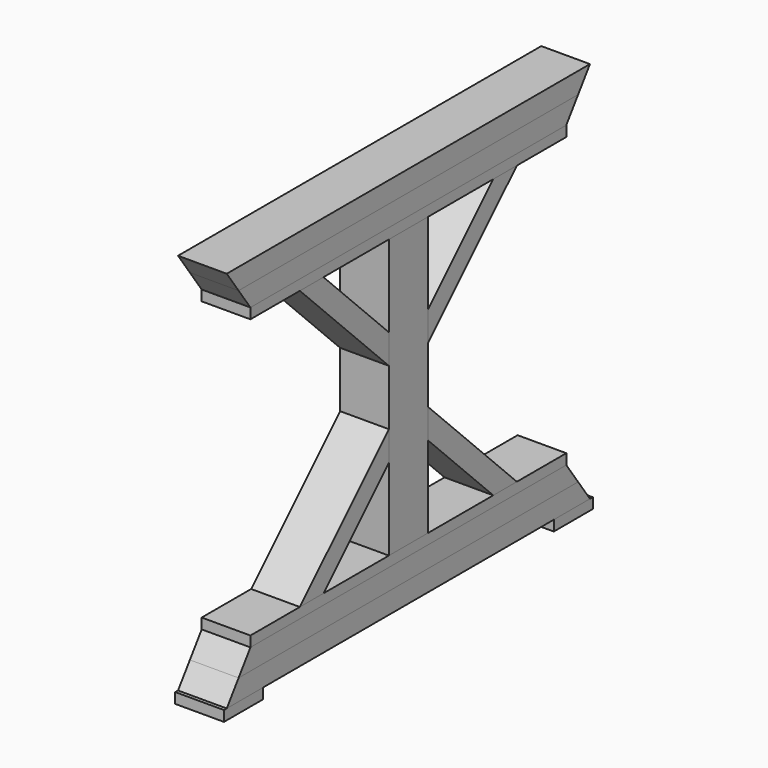
from build123d import *

# Parameters (mm, degrees)
F0_W      = 88.9
F0_H      = 38.1
F1_DEPTH  = 414.3375
F2_W      = 88.9
F2_H      = 38.1
F3_DEPTH  = 414.3375
F5_W      = 88.9
F5_H      = 19.05
F6_DEPTH  = 88.9
F8_W      = 88.9
F8_H      = 19.05
F9_DEPTH  = 360.3625
F11_DEPTH = 88.901
F12_W     = 88.9
F12_H     = 88.9
F13_DEPTH = 508
F17_DEPTH = 88.9


# Not quite as in the source:
# - a feature names something its author has since deleted; it is built from what else it names


with BuildPart() as f1:
    # F0 (on Front) → F1 (new body, symmetric)
    with BuildSketch(Plane.XZ):
        with Locations((44.45, 19.05)):
            Rectangle(F0_W, F0_H)
    extrude(amount=F1_DEPTH, both=True)


with BuildPart() as f3:
    # F2 (on Front) → F3 (new body, symmetric)
    with BuildSketch(Plane.XZ):
        with Locations((44.45, 57.15)):
            Rectangle(F2_W, F2_H)
    extrude(amount=F3_DEPTH, both=True)


with BuildPart() as f6:
    # F5 (on offset) → F6 (new body)
    with BuildSketch(Plane.XZ.offset(420.6875)):
        with Locations((44.45, -9.525)):
            Rectangle(F5_W, F5_H)
    extrude(amount=-F6_DEPTH)


with BuildPart() as f7_1:
    # F7: instance of F6
    add(f6.part.mirror(Plane.XZ))


with BuildPart() as f9:
    # F8 (on Front) → F9 (new body, symmetric)
    with BuildSketch(Plane.XZ):
        with Locations((44.45, 85.725)):
            Rectangle(F8_W, F8_H)
    extrude(amount=F9_DEPTH, both=True)


with BuildPart() as f11_tool:
    # F10 (on face) → F11 (new body, through all)
    with BuildSketch(Plane.YZ.offset(88.9)):
        Polygon((-360.300630331, 76.2), (-414.3375, 76.2), (-414.3375, 0), align=None)
        Polygon((360.300630331, 76.2), (414.3375, 0), (414.3375, 76.2), align=None)
    extrude(amount=-F11_DEPTH)


with BuildPart() as f1_1:
    add(f1.part)

    # F11: cut by f11_tool
    add(f11_tool.part, mode=Mode.SUBTRACT)


with BuildPart() as f3_1:
    add(f3.part)

    # F11: cut by f11_tool
    add(f11_tool.part, mode=Mode.SUBTRACT)


with BuildPart() as f13:
    # F12 (on face) → F13 (new body)
    with BuildSketch(Plane.XY.offset(95.25)):
        with Locations((44.45, 0)):
            Rectangle(F12_W, F12_H)
    extrude(amount=F13_DEPTH)


with BuildPart() as f15_1:
    # F15: instance of F9
    add(f9.part.mirror(Plane.XY.offset(349.25)))


with BuildPart() as f15_2:
    # F15: instance of F3
    add(f3_1.part.mirror(Plane.XY.offset(349.25)))


with BuildPart() as f15_3:
    # F15: instance of F1
    add(f1_1.part.mirror(Plane.XY.offset(349.25)))


with BuildPart() as f17:
    # F16 (on face) → F17 (new body)
    with BuildSketch(Plane(origin=(0, 0, 0), x_dir=(0, -1, 0), z_dir=(-1, 0, 0))):
        Polygon((-247.5565367264, 95.25), (-193.675, 95.25), (-44.45, 244.475), (-44.45, 298.3565367264), align=None)
    extrude(amount=-F17_DEPTH)


with BuildPart() as f18_1:
    # F18: instance of F17
    add(f17.part.mirror(Plane.XZ))


with BuildPart() as f19_1:
    # F19: instance of F17
    add(f17.part.mirror(Plane.XY.offset(349.25)))


with BuildPart() as f19_2:
    # F19: instance of F18_1
    add(f18_1.part.mirror(Plane.XY.offset(349.25)))


solid = Compound([f6.part, f7_1.part, f9.part, f1_1.part, f3_1.part, f13.part, f15_1.part, f15_2.part, f15_3.part, f17.part, f18_1.part, f19_1.part, f19_2.part])
